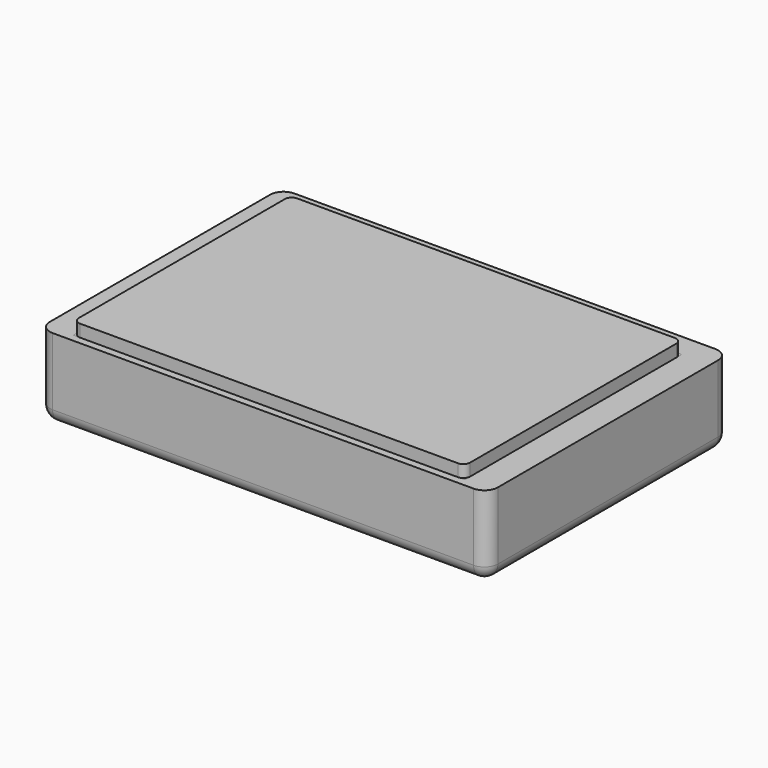
from build123d import *

# Parameters (mm, degrees)
F0_W     = 332
F0_H     = 224
F0_W_2   = 290
F0_H_2   = 201
F1_DEPTH = 60
F2_R     = 10
F3_DEPTH = 3
F4_DEPTH = 2.9
F5_DEPTH = 9.1
F6_R     = 5


# Not quite as in the source:
# - the program builds the solid bodies; features that only make, move or delete a surface that nothing else refers to are left out


with BuildPart() as f1:
    # F0 (on Top) → F1 (new body)
    with BuildSketch(Plane.XY):
        with Locations((0, 6)):
            Rectangle(F0_W, F0_H)
        Rectangle(F0_W_2, F0_H_2, mode=Mode.SUBTRACT)
        Rectangle(F0_W_2, F0_H_2)
    extrude(amount=-F1_DEPTH)

    # F2
    f2_edges = [f1.edges().sort_by_distance(p)[0] for p in [
        (166, -106, -30),
        (166, 118, -30),
        (-166, -106, -30),
        (0, -106, -60),
        (166, 6, -60),
        (-166, 6, -60),
        (0, 118, -60),
        (-166, 118, -30),
    ]]
    fillet(f2_edges, radius=F2_R)

    # F0 (on Top) → F3 (cut)
    with BuildSketch(Plane.XY):
        Rectangle(F0_W_2, F0_H_2)
    extrude(amount=-F3_DEPTH, mode=Mode.SUBTRACT)


with BuildPart() as f4:
    # F0 (on Top) → F4 (new body)
    with BuildSketch(Plane.XY):
        Rectangle(F0_W_2, F0_H_2)
    extrude(amount=-F4_DEPTH)


with BuildPart() as f5:
    # F0 (on Top) → F5 (new body)
    with BuildSketch(Plane.XY):
        Rectangle(F0_W_2, F0_H_2)
    extrude(amount=F5_DEPTH)

    # F6
    f6_edges = [f5.edges().sort_by_distance(p)[0] for p in [
        (145, -100.5, 4.55),
        (145, 100.5, 4.55),
        (-145, -100.5, 4.55),
        (-145, 100.5, 4.55),
    ]]
    fillet(f6_edges, radius=F6_R)


solid = Compound([f1.part, f4.part, f5.part])
